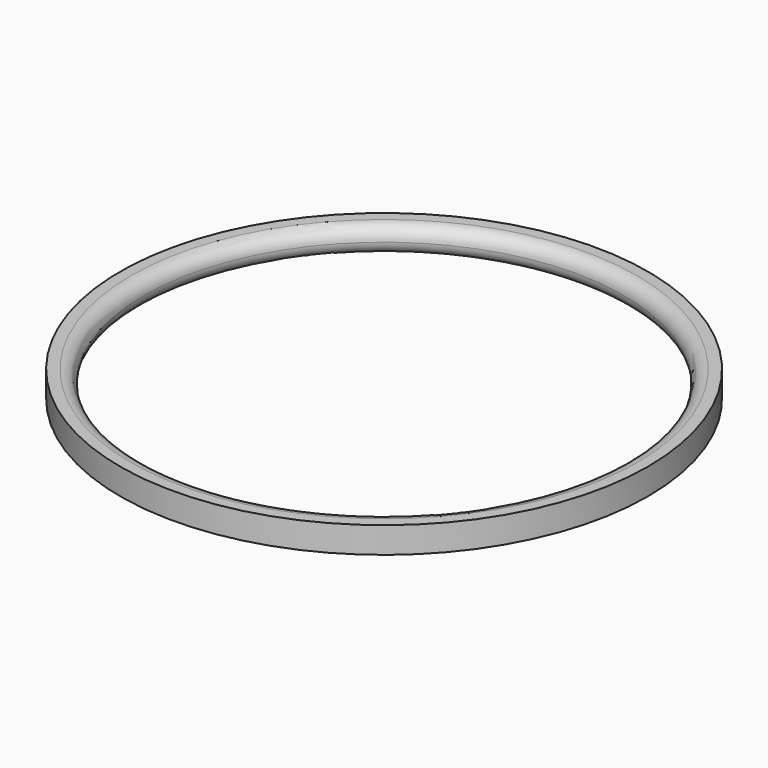
from build123d import *

# Parameters (mm, degrees)
F0_R     = 30.25
F0_R_2   = 27.5
F1_DEPTH = 3
F2_R     = 1.49999


# Not quite as in the source:
# - a fillet or chamfer is up to 0.001 mm smaller than in the source, because OpenCascade refuses the exact size


with BuildPart() as f1:
    # F0 (on Top) → F1 (new body)
    with BuildSketch(Plane.XY):
        Circle(F0_R)
        Circle(F0_R_2, mode=Mode.SUBTRACT)
    extrude(amount=F1_DEPTH)

    # F2 (radius 1.5 in the source; OpenCascade refuses exactly that, so slightly less here)
    f2_edges = [f1.edges().sort_by_distance(p)[0] for p in [
        (-27.5, 0, 3),
        (-27.5, 0, 0),
    ]]
    fillet(f2_edges, radius=F2_R)


solid = f1.part
